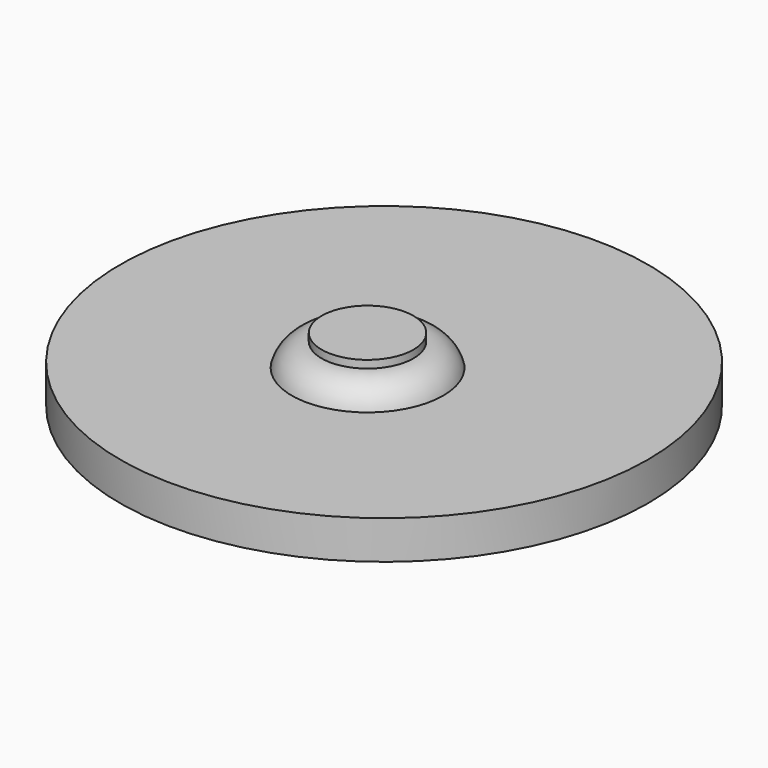
from build123d import *

# Parameters (mm, degrees)
F0_R     = 43.5689862092
F1_DEPTH = 6.35
F2_R     = 12.4962598147
F3_DEPTH = 3.81
F5_R     = 27.3162889884
F6_DEPTH = 1.27
F7_DEPTH = 1.27


# Not quite as in the source:
# - a fillet or chamfer that OpenCascade refuses, or shapes differently, is made with other operations: its cross-section is extruded or revolved along the edge and cut away or added


with BuildPart() as f1:
    # F0 (on Top) → F1 (new body)
    with BuildSketch(Plane.XY):
        Circle(F0_R)
    extrude(amount=F1_DEPTH)

    # F5 (on Top) → F6 (join)
    with BuildSketch(Plane.XY):
        with Locations((-0.5344543024, -1.2873198139)):
            Circle(F5_R)
    extrude(amount=-F6_DEPTH)


with BuildPart() as f3:
    # F2 (on face) → F3 (new body)
    with BuildSketch(Plane.XY.offset(6.35)):
        with Locations((-0.6934984121, -2.5477914605)):
            Circle(F2_R)
    extrude(amount=F3_DEPTH)

    # F4: fillet of radius 5.08 on 1 edges, made by hand

    # F4_s1 → F4_t2 (revolve, cut)
    with BuildSketch(Plane.XZ.offset(2.5477914605)):
        with BuildLine():
            ThreePointArc((11.8027614026, 6.35), (9.9949245263, 9.0960926284), (6.8840725529, 10.16))
            Line((6.8840725529, 10.16), (11.8027614026, 10.16))
            Line((11.8027614026, 10.16), (11.8027614026, 6.35))
        make_face()
    revolve(axis=Axis((-0.6934984121, -2.5477914605, 10.16), (0, 0, 1)), mode=Mode.SUBTRACT)

    # F7 (add): a face of the model
    f7_faces = [f3.faces().sort_by_distance(p)[0] for p in [
        (-0.6934984121, -2.5477914605, 10.16),
    ]]
    extrude(f7_faces, amount=F7_DEPTH)


solid = Compound([f1.part, f3.part])
